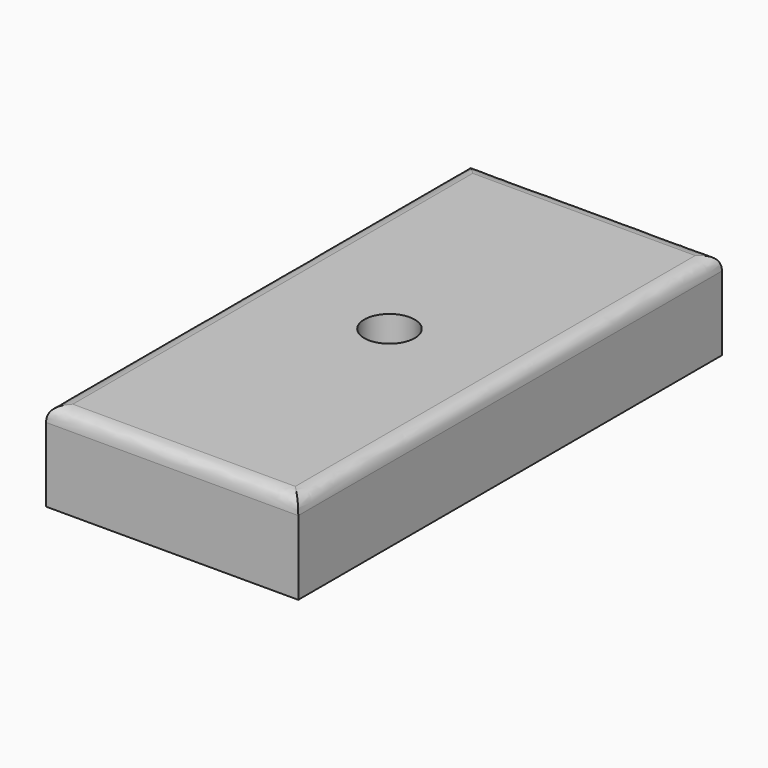
from build123d import *

# Parameters (mm, degrees)
F0_R          = 1.7
F1_DEPTH      = 1.5
F1_DEPTH_BACK = 6
F2_DEPTH      = 6
F3_T1_DEPTH   = 22
F3_T3_DEPTH   = 40.7


# Not quite as in the source:
# - a fillet or chamfer that OpenCascade refuses, or shapes differently, is made with other operations: its cross-section is extruded or revolved along the edge and cut away or added


with BuildPart() as f1:
    # F0 (on Top) → F1 (new body, two sides)
    with BuildSketch(Plane.XY) as f1_sk:
        Polygon((-4.7234346752, 0.4355579215), (-4.7234346752, -9.1929948391), (-2.7234009317, -14.6884420785), (2.9765315813, -14.6884420785), (4.9765653248, -9.1929948391), (4.9765653248, 0.4355579215), (4.9765653248, 10.028440195), (1.9944189816, 13.0115579215), (0.1265653248, 13.0115579215), (-1.7412883319, 13.0115579215), (-4.7234346752, 10.028440195), align=None)
        with Locations((0.1265653248, 0.4355579215)):
            Circle(F0_R, mode=Mode.SUBTRACT)
    extrude(amount=-F1_DEPTH)
    extrude(f1_sk.sketch, amount=F1_DEPTH_BACK)

    # F0 (on Top) → F2 (join)
    with BuildSketch(Plane.XY):
        Polygon((-8.5234346752, -17.6884420785), (0.1265653248, -17.6884420785), (4.9765653248, -17.6884420785), (8.4765653248, -17.6884420785), (8.4765653248, 18.0115579215), (-8.5234346752, 18.0115579215), align=None)
        Polygon((-2.7234009317, -14.6884420785), (-4.7234346752, -9.1929948391), (-4.7234346752, 0.4355579215), (-4.7234346752, 10.028440195), (-1.7412883319, 13.0115579215), (0.1265653248, 13.0115579215), (1.9944189816, 13.0115579215), (4.9765653248, 10.028440195), (4.9765653248, 0.4355579215), (4.9765653248, -9.1929948391), (2.9765315813, -14.6884420785), align=None, mode=Mode.SUBTRACT)
    extrude(amount=F2_DEPTH)

    # F3: fillet of radius 1 on 4 edges, made by hand

    # F3_s2 → F3_t1 (cut)
    with BuildSketch(Plane.YZ.offset(-11.0234346752)):
        with BuildLine():
            add(Edge.make_bspline(
                [(18.0115579215, 5), (18.0115579215, 6), (17.0115579215, 6)],
                knots=[0, 0, 0, 1, 1, 1], degree=2, weights=[1, 1, 1]))
            Line((17.0115579215, 6), (18.0115579215, 6))
            Line((18.0115579215, 6), (18.0115579215, 5))
        make_face()
        with BuildLine():
            add(Edge.make_bspline(
                [(-17.6884420785, 5), (-17.6884420785, 6), (-16.6884420785, 6)],
                knots=[0, 0, 0, 1, 1, 1], degree=2, weights=[1, 1, 1]))
            Line((-16.6884420785, 6), (-17.6884420785, 6))
            Line((-17.6884420785, 6), (-17.6884420785, 5))
        make_face()
    extrude(amount=F3_T1_DEPTH, mode=Mode.SUBTRACT)

    # F3_s4 → F3_t3 (cut)
    with BuildSketch(Plane.XZ.offset(-20.5115579215)):
        with BuildLine():
            add(Edge.make_bspline(
                [(-8.5234346752, 5), (-8.5234346752, 6), (-7.5234346752, 6)],
                knots=[0, 0, 0, 1, 1, 1], degree=2, weights=[1, 1, 1]))
            Line((-7.5234346752, 6), (-8.5234346752, 6))
            Line((-8.5234346752, 6), (-8.5234346752, 5))
        make_face()
        with BuildLine():
            add(Edge.make_bspline(
                [(8.4765653248, 5), (8.4765653248, 6), (7.4765653248, 6)],
                knots=[0, 0, 0, 1, 1, 1], degree=2, weights=[1, 1, 1]))
            Line((7.4765653248, 6), (8.4765653248, 6))
            Line((8.4765653248, 6), (8.4765653248, 5))
        make_face()
    extrude(amount=F3_T3_DEPTH, mode=Mode.SUBTRACT)


solid = f1.part
